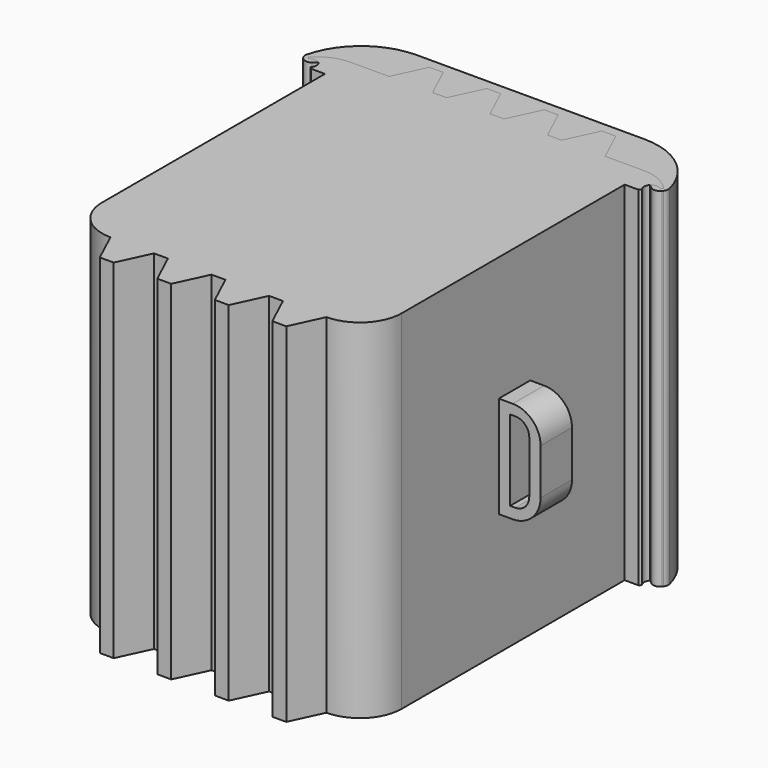
from build123d import *

# Parameters (mm, degrees)
F1_DEPTH     = 25
F2_W         = 18.5131066755
F2_H         = 22
F3_DEPTH     = 25
F4_W         = 2
F4_H         = 25
F5_DEPTH     = 2
F6_SIZE      = 1
F7_R         = 0.5
F8_DEPTH     = 25
F9_T1_DEPTH  = 36.1803398875
F11_DEPTH    = 0.5
F12_W        = 1.9662768522
F12_H        = 0.5
F12_W_2      = 0.5516889595
F13_DEPTH    = 0.5
F14_W        = 2.5179658116
F14_H        = 0.5
F15_DEPTH    = 0.5
F16_W        = 2.5179658116
F16_H        = 0.5
F17_DEPTH    = 0.5
F18_W        = 2.5179658116
F18_H        = 0.5
F19_DEPTH    = 0.5
F20_W        = 2.5179658116
F20_H        = 0.5
F21_W        = 2.5179658116
F21_H        = 0.5
F22_W        = 2.5179658116
F22_H        = 0.5
F23_W        = 2.5179658116
F23_H        = 0.5
F24_DEPTH    = 0.5
F25_W        = 1
F25_H        = 0.5
F26_DEPTH    = 0.5
F27_W        = 2.5179658116
F27_H        = 0.5
F28_W        = 3.2353515878
F28_H        = 0.5
F29_W        = 2.5179658116
F29_H        = 0.5
F30_W        = 2.5179658116
F30_H        = 0.5
F31_W        = 2.5179658116
F31_H        = 0.5
F32_W        = 2.5179658116
F32_H        = 0.5
F33_W        = 2.5179658116
F33_H        = 0.5
F34_W        = 2.5179658116
F34_H        = 0.5
F35_DEPTH    = 0.5
F36_W        = 1.906307787
F36_H        = 0.5
F36_W_2      = 1.7759219124
F36_W_3      = 2.08771969
F37_DEPTH    = 0.5
F39_DEPTH    = 25
F40_T1_DEPTH = 49.5481437958
F41_R        = 0.5
F42_W        = 2.8205653653
F42_H        = 7.3002856225
F43_DEPTH    = 3
F44_W        = 1.3718514529
F44_H        = 5.7771448046
F45_DEPTH    = 20
F46_R        = 2
F47_R        = 1
F48_R        = 2.99999


# Not quite as in the source:
# - a fillet or chamfer that OpenCascade refuses, or shapes differently, is made with other operations: its cross-section is extruded or revolved along the edge and cut away or added
# - a fillet or chamfer is up to 0.001 mm smaller than in the source, because OpenCascade refuses the exact size


with BuildPart() as f1:
    # F0 (on Top) → F1 (new body)
    with BuildSketch(Plane.XY):
        Polygon((-21.9865567995, 25), (-21.9865567995, 0), (-18.9865567995, 0), (-17.9224184651, -2.2820520226), (-16.9224184651, -2.2820520226), (-15.8582801306, 0), (-14.8582801306, 0), (-13.7941417962, -2.2820520226), (-12.7941417962, -2.2820520226), (-11.7300034618, 0), (-10.7300034618, 0), (-9.6658651273, -2.2820520226), (-8.6658651273, -2.2820520226), (-7.6017267929, 0), (-6.6017267929, 0), (-5.5375884584, -2.2820520226), (-4.5375884584, -2.2820520226), (-3.473450124, 0), (-0.473450124, 0), (-0.473450124, 25), (-3.473450124, 25), (-4.5375884584, 27.2820520226), (-5.5375884584, 27.2820520226), (-6.6017267929, 25), (-7.6017267929, 25), (-8.6658651273, 27.2820520226), (-9.6658651273, 27.2820520226), (-10.7300034618, 25), (-11.7300034618, 25), (-12.7941417962, 27.2820520226), (-13.7941417962, 27.2820520226), (-14.8582801306, 25), (-15.8582801306, 25), (-16.9224184651, 27.2820520226), (-17.9224184651, 27.2820520226), (-18.9865567995, 25), align=None)
    extrude(amount=F1_DEPTH)

    # F2 (on face) → F3 (cut)
    with BuildSketch(Plane(origin=(0, 27.2820520226, 0), x_dir=(-1, 0, 0), z_dir=(0, 1, 0))):
        with Locations((11.2300034618, 12.5)):
            Rectangle(F2_W, F2_H)
    extrude(amount=-F3_DEPTH, mode=Mode.SUBTRACT)

    # F4 (on face) → F5 (join)
    with BuildSketch(Plane(origin=(0, 25, 0), x_dir=(-1, 0, 0), z_dir=(0, 1, 0))):
        with Locations((-0.526549876, 12.5)):
            Rectangle(F4_W, F4_H)
        with Locations((22.9865567995, 12.5)):
            Rectangle(F4_W, F4_H)
    extrude(amount=-F5_DEPTH)

    # F6
    f6_edges = [f1.edges().sort_by_distance(p)[0] for p in [
        (1.52655, 23, 12.5),
        (-23.986557, 23, 12.5),
    ]]
    chamfer(f6_edges, length=F6_SIZE)

    # F7 (on face) → F8 (cut)
    with BuildSketch(Plane.XY.offset(25)):
        with Locations((1.026549876, 23.5)):
            Circle(F7_R)
        with Locations((-23.4865567995, 23.5)):
            Circle(F7_R)
    extrude(amount=-F8_DEPTH, mode=Mode.SUBTRACT)

    # F9: fillet of radius 3 on 2 edges, made by hand

    # F9_s2 → F9_t1 (cut)
    with BuildSketch(Plane.XY.offset(-5.5901699437)):
        with BuildLine():
            ThreePointArc((-23.9865567995, 24), (-22.9752336934, 24.7386127875), (-21.750488822, 25))
            Line((-21.750488822, 25), (-23.9865567995, 25))
            Line((-23.9865567995, 25), (-23.9865567995, 24))
        make_face()
        with BuildLine():
            ThreePointArc((-0.7095181015, 25), (0.5152267699, 24.7386127875), (1.526549876, 24))
            Line((1.526549876, 24), (1.526549876, 25))
            Line((1.526549876, 25), (-0.7095181015, 25))
        make_face()
    extrude(amount=F9_T1_DEPTH, mode=Mode.SUBTRACT)

    # F10 (on face) → F11 (cut)
    with BuildSketch(Plane(origin=(0, 27.2820520226, 0), x_dir=(-1, 0, 0), z_dir=(0, 1, 0))):
        Polygon((1.473450124, 1), (1.473450124, 24), (12.7941417962, 24), (12.7941417962, 24.5), (0.973450124, 24.5), (0.973450124, 0.5), (21.48652752, 0.5), (21.48652752, 24.5), (13.7941417962, 24.5), (13.7941417962, 24), (20.98652752, 24), (20.98652752, 1), align=None)
    extrude(amount=-F11_DEPTH, mode=Mode.SUBTRACT)

    # F12 (on face) → F13 (cut)
    with BuildSketch(Plane(origin=(6.7224851257, 3.1347462959, 0), x_dir=(-0.4226182617, 0.906307787, 0), z_dir=(0.906307787, 0.4226182617, 0))):
        with Locations((25.1087765556, 0.75)):
            Rectangle(F12_W, F12_H)
        with Locations((26.3677594615, 0.75)):
            Rectangle(F12_W_2, F12_H)
    extrude(amount=-F13_DEPTH, mode=Mode.SUBTRACT)

    # F14 (on face) → F15 (cut)
    with BuildSketch(Plane(origin=(3.3315442452, 1.553524595, 0), x_dir=(-0.4226182617, 0.906307787, 0), z_dir=(0.906307787, 0.4226182617, 0))):
        with Locations((27.5585632771, 0.75)):
            Rectangle(F14_W, F14_H)
    extrude(amount=-F15_DEPTH, mode=Mode.SUBTRACT)

    # F16 (on face) → F17 (cut)
    with BuildSketch(Plane(origin=(-0.0593966353, -0.0276971059, 0), x_dir=(-0.4226182617, 0.906307787, 0), z_dir=(0.906307787, 0.4226182617, 0))):
        with Locations((28.5654719919, 0.75)):
            Rectangle(F16_W, F16_H)
    extrude(amount=-F17_DEPTH, mode=Mode.SUBTRACT)

    # F18 (on face) → F19 (cut)
    with BuildSketch(Plane(origin=(-3.4503375158, -1.6089188068, 0), x_dir=(-0.4226182617, 0.906307787, 0), z_dir=(0.906307787, 0.4226182617, 0))):
        with Locations((30.6186763647, 0.75)):
            Rectangle(F18_W, F18_H)
    extrude(amount=-F19_DEPTH, mode=Mode.SUBTRACT)

    # F20 (on face) + F21 (on face) + F22 (on face) + F23 (on face) → F24 (cut)
    with BuildSketch(Plane(origin=(6.7224851257, 3.1347462959, 0), x_dir=(-0.4226182617, 0.906307787, 0), z_dir=(0.906307787, 0.4226182617, 0))):
        with Locations((25.3846210354, 24.25)):
            Rectangle(F20_W, F20_H)
    with BuildSketch(Plane(origin=(3.3315442452, 1.553524595, 0), x_dir=(-0.4226182617, 0.906307787, 0), z_dir=(0.906307787, 0.4226182617, 0))):
        with Locations((27.1293061452, 24.25)):
            Rectangle(F21_W, F21_H)
    with BuildSketch(Plane(origin=(-0.0593966353, -0.0276971059, 0), x_dir=(-0.4226182617, 0.906307787, 0), z_dir=(0.906307787, 0.4226182617, 0))):
        with Locations((28.873991255, 24.25)):
            Rectangle(F22_W, F22_H)
    with BuildSketch(Plane(origin=(-3.4503375158, -1.6089188068, 0), x_dir=(-0.4226182617, 0.906307787, 0), z_dir=(0.906307787, 0.4226182617, 0))):
        with Locations((30.6186763647, 24.25)):
            Rectangle(F23_W, F23_H)
    extrude(amount=-F24_DEPTH, mode=Mode.SUBTRACT)

    # F25 (on face) → F26 (cut)
    with BuildSketch(Plane(origin=(0, 27.2820520226, 0), x_dir=(-1, 0, 0), z_dir=(0, 1, 0))):
        with Locations((13.2941417962, 24.25)):
            Rectangle(F25_W, F25_H)
    extrude(amount=-F26_DEPTH, mode=Mode.SUBTRACT)

    # F27 (on face) + F28 (on face) + F29 (on face) + F30 (on face) + F31 (on face) + F32 (on face) + F33 (on face) + F34 (on face) → F35 (cut)
    with BuildSketch(Plane(origin=(-14.9981730279, 6.9937629413, 0), x_dir=(-0.4226182617, -0.906307787, 0), z_dir=(-0.906307787, 0.4226182617, 0))):
        with Locations((-21.12666728, 0.75)):
            Rectangle(F27_W, F27_H)
    with BuildSketch(Plane(origin=(-18.3891139084, 8.5749846422, 0), x_dir=(-0.4226182617, -0.906307787, 0), z_dir=(-0.906307787, 0.4226182617, 0))):
        with Locations((-19.7406750583, 0.75)):
            Rectangle(F28_W, F28_H)
    with BuildSketch(Plane(origin=(-21.7800547889, 10.1562063431, 0), x_dir=(-0.4226182617, -0.906307787, 0), z_dir=(-0.906307787, 0.4226182617, 0))):
        with Locations((-17.6372970605, 0.75)):
            Rectangle(F29_W, F29_H)
    with BuildSketch(Plane(origin=(-25.1709956694, 11.737428044, 0), x_dir=(-0.4226182617, -0.906307787, 0), z_dir=(-0.906307787, 0.4226182617, 0))):
        with Locations((-15.8926119507, 0.75)):
            Rectangle(F30_W, F30_H)
    with BuildSketch(Plane(origin=(-25.1709956694, 11.737428044, 0), x_dir=(-0.4226182617, -0.906307787, 0), z_dir=(-0.906307787, 0.4226182617, 0))):
        with Locations((-15.8926119507, 24.25)):
            Rectangle(F31_W, F31_H)
    with BuildSketch(Plane(origin=(-21.7800547889, 10.1562063431, 0), x_dir=(-0.4226182617, -0.906307787, 0), z_dir=(-0.906307787, 0.4226182617, 0))):
        with Locations((-17.6372970605, 24.25)):
            Rectangle(F32_W, F32_H)
    with BuildSketch(Plane(origin=(-18.3891139084, 8.5749846422, 0), x_dir=(-0.4226182617, -0.906307787, 0), z_dir=(-0.906307787, 0.4226182617, 0))):
        with Locations((-19.3819821703, 24.25)):
            Rectangle(F33_W, F33_H)
    with BuildSketch(Plane(origin=(-14.9981730279, 6.9937629413, 0), x_dir=(-0.4226182617, -0.906307787, 0), z_dir=(-0.906307787, 0.4226182617, 0))):
        with Locations((-21.12666728, 24.25)):
            Rectangle(F34_W, F34_H)
    extrude(amount=-F35_DEPTH, mode=Mode.SUBTRACT)

    # F36 (on face) → F37 (cut)
    with BuildSketch(Plane(origin=(0, 25, 0), x_dir=(-1, 0, 0), z_dir=(0, 1, 0))):
        Polygon((1.473450124, 1), (1.473450124, 24), (3.9266040175, 24), (3.9266040175, 24.5), (0.973450124, 24.5), (0.973450124, 0.5), (3.9266040175, 0.5), (3.9266040175, 1), align=None)
        Polygon((18.533402906, 24), (20.9865567995, 24), (20.9865567995, 1), (18.533402906, 1), (18.533402906, 0.5), (21.4865567995, 0.5), (21.4865567995, 24.5), (18.533402906, 24.5), align=None)
        with Locations((15.3582801306, 0.75)):
            Rectangle(F36_W, F36_H)
        with Locations((11.1648105244, 0.75)):
            Rectangle(F36_W_2, F36_H)
        with Locations((7.1924327444, 0.75)):
            Rectangle(F36_W_3, F36_H)
        with Locations((7.1017267929, 24.25)):
            Rectangle(F36_W, F36_H)
        with Locations((11.2300034618, 24.25)):
            Rectangle(F36_W, F36_H)
        with Locations((15.3582801306, 24.25)):
            Rectangle(F36_W, F36_H)
    extrude(amount=-F37_DEPTH, mode=Mode.SUBTRACT)

    # F42 (on face) → F43 (join)
    with BuildSketch(Plane.YZ.offset(-0.473450124)):
        with Locations((13.1176770665, 12.4170416966)):
            Rectangle(F42_W, F42_H)
    extrude(amount=F43_DEPTH)

    # F44 (on face) → F45 (cut)
    with BuildSketch(Plane(origin=(0, 14.5279597491, 0), x_dir=(-1, 0, 0), z_dir=(0, 1, 0))):
        with Locations((-1.0279472772, 12.4440519139)):
            Rectangle(F44_W, F44_H)
    extrude(amount=-F45_DEPTH, mode=Mode.SUBTRACT)

    # F46
    f46_edges = [f1.edges().sort_by_distance(p)[0] for p in [
        (2.52655, 13.117677, 8.766899),
        (2.52655, 13.117677, 16.067185),
    ]]
    fillet(f46_edges, radius=F46_R)

    # F47
    f47_edges = [f1.edges().sort_by_distance(p)[0] for p in [
        (1.713873, 13.117677, 15.332624),
        (1.713873, 13.117677, 9.55548),
    ]]
    fillet(f47_edges, radius=F47_R)

    # F48 (radius 3 in the source; OpenCascade refuses exactly that, so slightly less here)
    f48_edges = [f1.edges().sort_by_distance(p)[0] for p in [
        (-0.47345, 0, 12.5),
        (-21.986557, 0, 12.5),
    ]]
    fillet(f48_edges, radius=F48_R)


with BuildPart() as f39:
    # F38 (on face) → F39 (new body)
    with BuildSketch(Plane.XY.offset(25)):
        with BuildLine():
            ThreePointArc((-23.9865567995, 24), (-22.9752336934, 24.7386127875), (-21.750488822, 25))
            Line((-21.750488822, 25), (-18.9865567995, 25))
            Line((-18.9865567995, 25), (-17.9224184651, 27.2820520226))
            Line((-17.9224184651, 27.2820520226), (-16.9224184651, 27.2820520226))
            Line((-16.9224184651, 27.2820520226), (-15.8582801306, 25))
            Line((-15.8582801306, 25), (-14.8582801306, 25))
            Line((-14.8582801306, 25), (-13.7941417962, 27.2820520226))
            Line((-13.7941417962, 27.2820520226), (-12.7941417962, 27.2820520226))
            Line((-12.7941417962, 27.2820520226), (-11.7300034618, 25))
            Line((-11.7300034618, 25), (-10.7300034618, 25))
            Line((-10.7300034618, 25), (-9.6658651273, 27.2820520226))
            Line((-9.6658651273, 27.2820520226), (-8.6658651273, 27.2820520226))
            Line((-8.6658651273, 27.2820520226), (-7.6017267929, 25))
            Line((-7.6017267929, 25), (-6.6017267929, 25))
            Line((-6.6017267929, 25), (-5.5375884584, 27.2820520226))
            Line((-5.5375884584, 27.2820520226), (-4.5375884584, 27.2820520226))
            Line((-4.5375884584, 27.2820520226), (-3.473450124, 25))
            Line((-3.473450124, 25), (-0.7095181015, 25))
            ThreePointArc((-0.7095181015, 25), (0.5152267699, 24.7386127875), (1.526549876, 24))
            Line((1.526549876, 24), (1.3801032666, 23.8535533906))
            ThreePointArc((1.3801032666, 23.8535533906), (1.026549876, 24), (0.6729964854, 23.8535533906))
            Line((0.6729964854, 23.8535533906), (1.3372162357, 23.3178287745))
            Line((1.3372162357, 23.3178287745), (1.8441342952, 23.9463326303))
            Line((1.8441342952, 23.9463326303), (1.8441342952, 28))
            Line((1.8441342952, 28), (-24.3041412188, 28))
            Line((-24.3041412188, 28), (-24.3041412188, 23.9463326303))
            Line((-24.3041412188, 23.9463326303), (-23.7972231592, 23.3178287745))
            Line((-23.7972231592, 23.3178287745), (-23.1330034089, 23.8535533906))
            ThreePointArc((-23.1330034089, 23.8535533906), (-23.4865567995, 24), (-23.8401101901, 23.8535533906))
            Line((-23.8401101901, 23.8535533906), (-23.9865567995, 24))
        make_face()
    extrude(amount=-F39_DEPTH)

    # F40: fillet of radius 5 on 2 edges, made by hand

    # F40_s2 → F40_t1 (cut)
    with BuildSketch(Plane.XY.offset(-12.2740718979)):
        with BuildLine():
            ThreePointArc((1.8441342952, 23.9463326303), (0.1179264043, 26.8556233706), (-3.0654944639, 28))
            Line((-3.0654944639, 28), (1.8441342952, 28))
            Line((1.8441342952, 28), (1.8441342952, 23.9463326303))
        make_face()
        with BuildLine():
            ThreePointArc((-19.3945124596, 28), (-22.5779333278, 26.8556233706), (-24.3041412188, 23.9463326303))
            Line((-24.3041412188, 23.9463326303), (-24.3041412188, 28))
            Line((-24.3041412188, 28), (-19.3945124596, 28))
        make_face()
    extrude(amount=F40_T1_DEPTH, mode=Mode.SUBTRACT)

    # F41
    f41_edges = [f39.edges().sort_by_distance(p)[0] for p in [
        (1.337216, 23.317829, 12.5),
        (1.844134, 23.946333, 12.5),
        (-24.304141, 23.946333, 12.5),
        (-23.797223, 23.317829, 12.5),
    ]]
    fillet(f41_edges, radius=F41_R)


solid = Compound([f1.part, f39.part])
